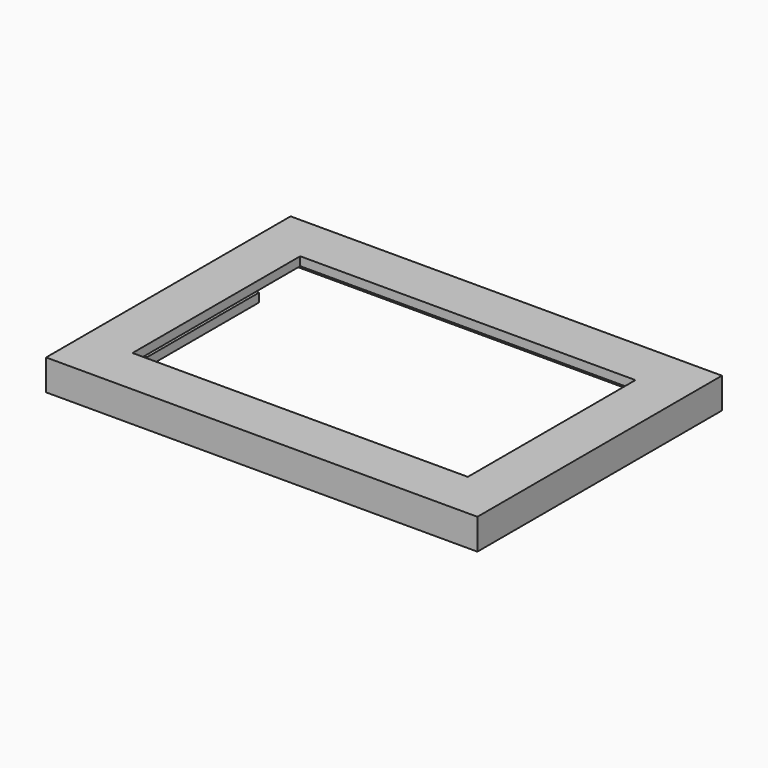
from build123d import *

# Parameters (mm, degrees)
F0_W      = 156.845
F0_H      = 111.125
F0_W_2    = 1.5875
F0_H_2    = 50.8
F1_DEPTH  = 8
F0_W_3    = 6.35
F0_R      = 1.5875
F2_DEPTH  = 3.175
F3_W      = 156.845
F3_H      = 111.125
F3_W_2    = 144.145
F3_H_2    = 98.425
F3_W_3    = 121.92
F3_H_3    = 76.2
F4_DEPTH  = 3.175
F5_R      = 1.5875
F6_W      = 101.6
F6_H      = 1.5875
F7_DEPTH  = 9.525
F8_W      = 6.35
F8_H      = 1.5875
F9_DEPTH  = 4.7625
F10_DEPTH = 1.5875
F11_DEPTH = 2.38125


with BuildPart() as f1:
    # F0 (on Top) → F1 (new body)
    with BuildSketch(Plane.XY):
        Rectangle(F0_W, F0_H)
        with BuildLine():
            Line((75.2475, -53.975), (-75.2475, -53.975))
            ThreePointArc((-75.2475, -53.975), (-76.3700320151, -53.5100320151), (-76.835, -52.3875))
            Line((-76.835, -52.3875), (-76.835, 52.3875))
            ThreePointArc((-76.835, 52.3875), (-76.3700320151, 53.5100320151), (-75.2475, 53.975))
            Line((-75.2475, 53.975), (75.2475, 53.975))
            ThreePointArc((75.2475, 53.975), (76.3700320151, 53.5100320151), (76.835, 52.3875))
            Line((76.835, 52.3875), (76.835, -52.3875))
            ThreePointArc((76.835, -52.3875), (76.3700320151, -53.5100320151), (75.2475, -53.975))
        make_face(mode=Mode.SUBTRACT)
        with BuildLine():
            ThreePointArc((-76.835, -52.3875), (-76.3700320151, -53.5100320151), (-75.2475, -53.975))
            Line((-75.2475, -53.975), (75.2475, -53.975))
            ThreePointArc((75.2475, -53.975), (76.3700320151, -53.5100320151), (76.835, -52.3875))
            Line((76.835, -52.3875), (76.835, 52.3875))
            ThreePointArc((76.835, 52.3875), (76.3700320151, 53.5100320151), (75.2475, 53.975))
            Line((75.2475, 53.975), (-75.2475, 53.975))
            ThreePointArc((-75.2475, 53.975), (-76.3700320151, 53.5100320151), (-76.835, 52.3875))
            Line((-76.835, 52.3875), (-76.835, -52.3875))
        make_face()
        with BuildLine():
            ThreePointArc((-73.66, 49.2125), (-73.1950320151, 50.3350320151), (-72.0725, 50.8))
            Line((-72.0725, 50.8), (72.0725, 50.8))
            ThreePointArc((72.0725, 50.8), (73.1950320151, 50.3350320151), (73.66, 49.2125))
            Line((73.66, 49.2125), (73.66, 25.4))
            Line((73.66, 25.4), (73.66, -25.4))
            Line((73.66, -25.4), (73.66, -49.2125))
            ThreePointArc((73.66, -49.2125), (73.1950320151, -50.3350320151), (72.0725, -50.8))
            Line((72.0725, -50.8), (-72.0725, -50.8))
            ThreePointArc((-72.0725, -50.8), (-73.1950320151, -50.3350320151), (-73.66, -49.2125))
            Line((-73.66, -49.2125), (-73.66, -25.4))
            Line((-73.66, -25.4), (-73.66, 25.4))
            Line((-73.66, 25.4), (-73.66, 49.2125))
        make_face(mode=Mode.SUBTRACT)
        with BuildLine():
            Line((-72.0725, -25.4), (-73.66, -25.4))
            Line((-73.66, -25.4), (-73.66, -49.2125))
            ThreePointArc((-73.66, -49.2125), (-73.1950320151, -50.3350320151), (-72.0725, -50.8))
            Line((-72.0725, -50.8), (72.0725, -50.8))
            ThreePointArc((72.0725, -50.8), (73.1950320151, -50.3350320151), (73.66, -49.2125))
            Line((73.66, -49.2125), (73.66, -25.4))
            Line((73.66, -25.4), (72.0725, -25.4))
            Line((72.0725, -25.4), (72.0725, -49.2125))
            Line((72.0725, -49.2125), (-72.0725, -49.2125))
            Line((-72.0725, -49.2125), (-72.0725, -25.4))
        make_face()
        with BuildLine():
            Line((72.0725, 50.8), (-72.0725, 50.8))
            ThreePointArc((-72.0725, 50.8), (-73.1950320151, 50.3350320151), (-73.66, 49.2125))
            Line((-73.66, 49.2125), (-73.66, 25.4))
            Line((-73.66, 25.4), (-72.0725, 25.4))
            Line((-72.0725, 25.4), (-72.0725, 49.2125))
            Line((-72.0725, 49.2125), (72.0725, 49.2125))
            Line((72.0725, 49.2125), (72.0725, 25.4))
            Line((72.0725, 25.4), (73.66, 25.4))
            Line((73.66, 25.4), (73.66, 49.2125))
            ThreePointArc((73.66, 49.2125), (73.1950320151, 50.3350320151), (72.0725, 50.8))
        make_face()
        with Locations((-72.86625, 0)):
            Rectangle(F0_W_2, F0_H_2)
        with Locations((72.86625, 0)):
            Rectangle(F0_W_2, F0_H_2)
    extrude(amount=F1_DEPTH)

    # F0 (on Top) → F2 (join)
    with BuildSketch(Plane.XY):
        with Locations((68.8975, 0)):
            Rectangle(F0_W_3, F0_H_2)
        with Locations((69.05625, -15.875)):
            Circle(F0_R, mode=Mode.SUBTRACT)
        with Locations((69.05625, 15.875)):
            Circle(F0_R, mode=Mode.SUBTRACT)
        with Locations((-68.8975, 0)):
            Rectangle(F0_W_3, F0_H_2)
        with Locations((-69.05625, -15.875)):
            Circle(F0_R, mode=Mode.SUBTRACT)
        with Locations((-69.05625, 15.875)):
            Circle(F0_R, mode=Mode.SUBTRACT)
    extrude(amount=F2_DEPTH)

    # F3 (on face) → F4 (join)
    with BuildSketch(Plane.XY.offset(8)):
        Rectangle(F3_W, F3_H)
        Rectangle(F3_W_2, F3_H_2, mode=Mode.SUBTRACT)
        Rectangle(F3_W_2, F3_H_2)
        Rectangle(F3_W_3, F3_H_3, mode=Mode.SUBTRACT)
    extrude(amount=F4_DEPTH)

    # F5
    f5_edges = [f1.edges().sort_by_distance(p)[0] for p in [
        (-72.0725, -49.2125, 4),
        (-72.0725, 49.2125, 4),
        (72.0725, -49.2125, 4),
        (72.0725, 49.2125, 4),
    ]]
    fillet(f5_edges, radius=F5_R)

    # F6 (on face) → F7 (join)
    with BuildSketch(Plane(origin=(0, -49.2125, 0), x_dir=(-1, 0, 0), z_dir=(0, 1, 0))):
        with Locations((0, 4.70625)):
            Rectangle(F6_W, F6_H)
    extrude(amount=F7_DEPTH)

    # F8 (on face) → F9 (join)
    with BuildSketch(Plane.XZ.offset(-49.2125)):
        with Locations((-34.925, 4.70625)):
            Rectangle(F8_W, F8_H)
        with Locations((34.925, 4.70625)):
            Rectangle(F8_W, F8_H)
    extrude(amount=F9_DEPTH)

    # F0 (on Top) → F10 (cut)
    with BuildSketch(Plane.XY):
        with BuildLine():
            ThreePointArc((-76.835, -52.3875), (-76.3700320151, -53.5100320151), (-75.2475, -53.975))
            Line((-75.2475, -53.975), (75.2475, -53.975))
            ThreePointArc((75.2475, -53.975), (76.3700320151, -53.5100320151), (76.835, -52.3875))
            Line((76.835, -52.3875), (76.835, 52.3875))
            ThreePointArc((76.835, 52.3875), (76.3700320151, 53.5100320151), (75.2475, 53.975))
            Line((75.2475, 53.975), (-75.2475, 53.975))
            ThreePointArc((-75.2475, 53.975), (-76.3700320151, 53.5100320151), (-76.835, 52.3875))
            Line((-76.835, 52.3875), (-76.835, -52.3875))
        make_face()
        with BuildLine():
            ThreePointArc((-73.66, 49.2125), (-73.1950320151, 50.3350320151), (-72.0725, 50.8))
            Line((-72.0725, 50.8), (72.0725, 50.8))
            ThreePointArc((72.0725, 50.8), (73.1950320151, 50.3350320151), (73.66, 49.2125))
            Line((73.66, 49.2125), (73.66, 25.4))
            Line((73.66, 25.4), (73.66, -25.4))
            Line((73.66, -25.4), (73.66, -49.2125))
            ThreePointArc((73.66, -49.2125), (73.1950320151, -50.3350320151), (72.0725, -50.8))
            Line((72.0725, -50.8), (-72.0725, -50.8))
            ThreePointArc((-72.0725, -50.8), (-73.1950320151, -50.3350320151), (-73.66, -49.2125))
            Line((-73.66, -49.2125), (-73.66, -25.4))
            Line((-73.66, -25.4), (-73.66, 25.4))
            Line((-73.66, 25.4), (-73.66, 49.2125))
        make_face(mode=Mode.SUBTRACT)
    extrude(amount=F10_DEPTH, mode=Mode.SUBTRACT)


with BuildPart() as f11:
    # F11 (new): a face of the model
    f11_faces = [f1.part.faces().sort_by_distance(p)[0] for p in [
        (-75.0421074804, 52.1821074804, 1.5875),
    ]]
    extrude(f11_faces, amount=F11_DEPTH)


solid = Compound([f1.part, f11.part])
